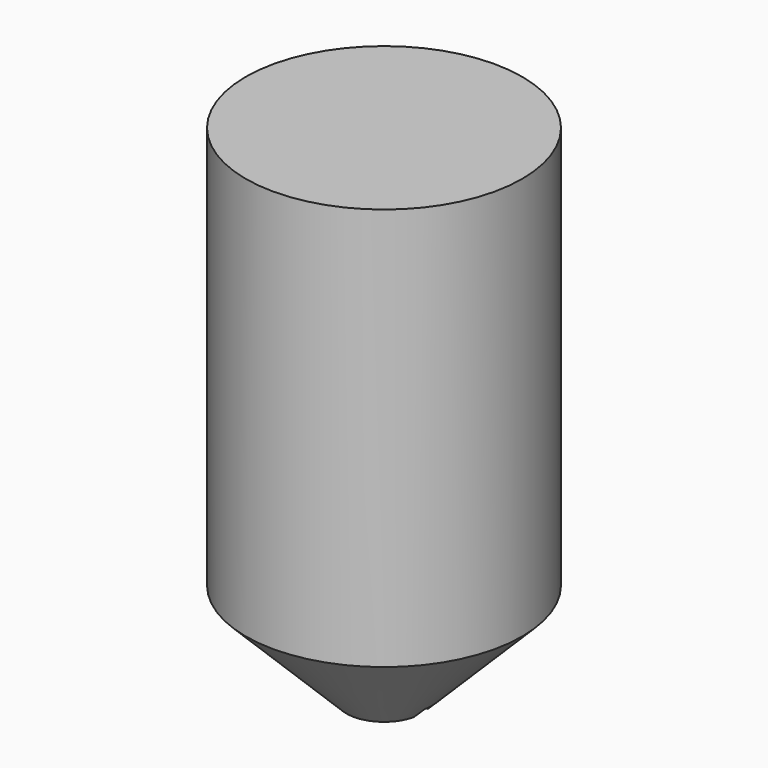
from build123d import *
from build123d import SkipClean  # not in build123d's __all__

# Parameters (mm, degrees)
F0_R       = 34.8665776849
F1_DEPTH   = 127
F2_SIZE    = 25.4
F3_W       = 0.0296507081
F3_H       = 2.1137676667
F3_W_2     = 1.5040034195
F3_H_2     = 6.3516600603
F3_W_3     = 5.515434417
F1_FACE_R  = 9.4665776849
F1_FACE1_R = 34.8665776849
F4_DEPTH   = 76.2


with BuildPart() as f1:
    # F0 (on Top) → F1 (new body)
    with BuildSketch(Plane.XY):
        Circle(F0_R)
    extrude(amount=F1_DEPTH)

    # F2
    f2_edges = [f1.edges().sort_by_distance(p)[0] for p in [
        (-34.866578, 0, 0),
    ]]
    chamfer(f2_edges, length=F2_SIZE)

    # F3 (on face) + F1_face (on face) + F1_face1 (on face) → F4 (cut)
    with BuildSketch(Plane(origin=(0, 0, 0), x_dir=(1, 0, 0), z_dir=(0, 0, -1))):
        with Locations((7.0046124826, 1.0568838334)):
            Rectangle(F3_W, F3_H)
        with Locations((7.0046124826, -1.0568838334)):
            Rectangle(F3_W, F3_H)
        with Locations((0.7520017098, -3.1758300302)):
            Rectangle(F3_W_2, F3_H_2)
        with BuildLine():
            Line((7.0194378366, 2.1137676667), (7.0194378366, 0))
            Line((7.0194378366, 0), (9.4665776849, 0))
            ThreePointArc((9.4665776849, 0), (9.4066364158, 1.0636185423), (9.2275716911, 2.1137676667))
            Line((9.2275716911, 2.1137676667), (7.0194378366, 2.1137676667))
        make_face()
        with BuildLine():
            Line((7.0194378366, 0), (7.0194378366, -2.1137676667))
            Line((7.0194378366, -2.1137676667), (9.2275716911, -2.1137676667))
            ThreePointArc((9.2275716911, -2.1137676667), (9.4066364158, -1.0636185423), (9.4665776849, 0))
            Line((9.4665776849, 0), (7.0194378366, 0))
        make_face()
        with BuildLine():
            ThreePointArc((9.4665776849, 0), (9.4066364158, -1.0636185423), (9.2275716911, -2.1137676667))
            Line((9.2275716911, -2.1137676667), (11.9433682412, -2.1137676667))
            Line((11.9433682412, -2.1137676667), (11.9433682412, 2.1137676667))
            Line((11.9433682412, 2.1137676667), (9.2275716911, 2.1137676667))
            ThreePointArc((9.2275716911, 2.1137676667), (9.4066364158, 1.0636185423), (9.4665776849, 0))
        make_face()
        with Locations((-4.2617206281, 3.1758300302)):
            Rectangle(F3_W_3, F3_H_2)
        with Locations((-4.2617206281, -3.1758300302)):
            Rectangle(F3_W_3, F3_H_2)
        Polygon((1.5040034195, -6.3516600603), (7.0194378366, -6.3516600603), (7.0194378366, -2.1137676667), (6.9897871285, -2.1137676667), (6.9897871285, 0), (1.5040034195, 0), align=None)
        Polygon((1.5040034195, 6.3516600603), (1.5040034195, 0), (6.9897871285, 0), (6.9897871285, 2.1137676667), (7.0194378366, 2.1137676667), (7.0194378366, 6.3516600603), align=None)
        with Locations((0.7520017098, 3.1758300302)):
            Rectangle(F3_W_2, F3_H_2)
        with Locations((-0.7520017098, 3.1758300302)):
            Rectangle(F3_W_2, F3_H_2)
        with BuildLine():
            Line((-1.5040034195, 6.3516600603), (0, 6.3516600603))
            Line((0, 6.3516600603), (0, 9.4665776849))
            ThreePointArc((0, 9.4665776849), (-3.8397662477, 8.6528774535), (-7.0194378366, 6.3516600603))
            Line((-7.0194378366, 6.3516600603), (-1.5040034195, 6.3516600603))
        make_face()
        with Locations((-0.7520017098, -3.1758300302)):
            Rectangle(F3_W_2, F3_H_2)
        with BuildLine():
            Line((0, 9.4665776849), (0, 6.3516600603))
            Line((0, 6.3516600603), (1.5040034195, 6.3516600603))
            Line((1.5040034195, 6.3516600603), (7.0194378366, 6.3516600603))
            ThreePointArc((7.0194378366, 6.3516600603), (3.8397662477, 8.6528774535), (0, 9.4665776849))
        make_face()
        with BuildLine():
            Line((0, -6.3516600603), (0, -9.4665776849))
            ThreePointArc((0, -9.4665776849), (3.8397662477, -8.6528774535), (7.0194378366, -6.3516600603))
            Line((7.0194378366, -6.3516600603), (1.5040034195, -6.3516600603))
            Line((1.5040034195, -6.3516600603), (0, -6.3516600603))
        make_face()
    with BuildSketch(Plane(origin=(0, 0, 0), x_dir=(1, 0, 0), z_dir=(0, 0, -1))):
        Circle(F1_FACE_R)
    with BuildSketch(Plane.XY.offset(127)):
        Circle(F1_FACE1_R)
    extrude(amount=-F4_DEPTH, dir=(0, 0, -1), mode=Mode.SUBTRACT)

    # F5: F1 across plane


with BuildPart() as f1_1:
    add(f1.part, clean=False)
    with SkipClean():  # cleaning this boolean's faces spoils the solid; the shape is the same uncleaned
        add(f1.part.mirror(Plane.XZ), clean=False)


solid = f1_1.part
